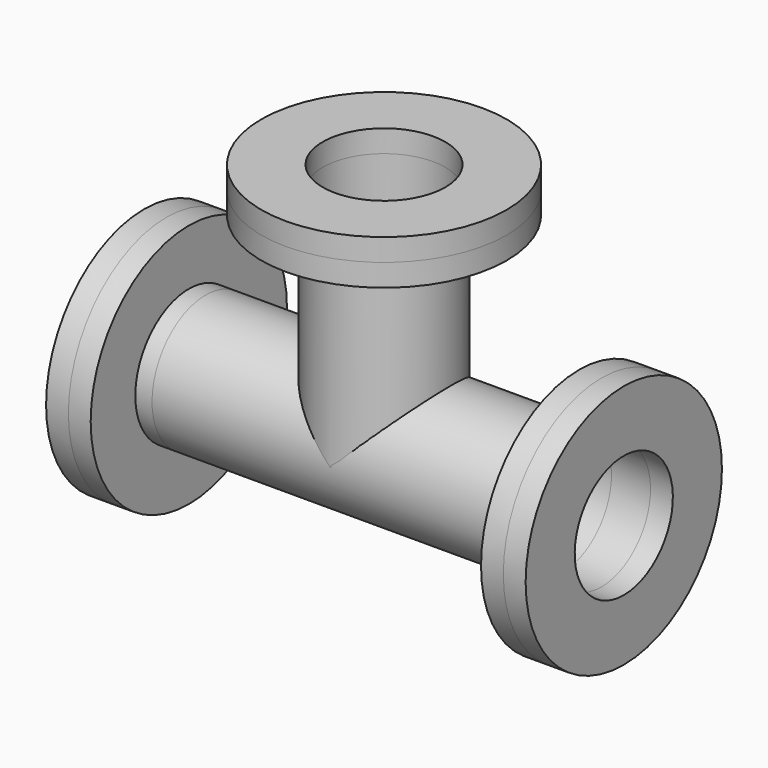
from build123d import *

# Parameters (mm, degrees)
F0_R      = 76.2
F0_R_2    = 69.85
F1_DEPTH  = 19.05
F2_R      = 139.7
F2_R_2    = 76.2
F2_R_3    = 69.85
F3_DEPTH  = 25.4
F9_ANGLE  = 90
F11_DEPTH = 406.4
F12_REACH = 558.4271469057
F13_DEPTH = 25.4
F14_DEPTH = 25.4
F15_DEPTH = 25.4


with BuildPart() as f1:
    # F0 (on Top) → F1 (new body)
    with BuildSketch(Plane.XY):
        Circle(F0_R)
        Circle(F0_R_2, mode=Mode.SUBTRACT)
    extrude(amount=F1_DEPTH)

    # F2 (on face) → F3 (join)
    with BuildSketch(Plane.XY.offset(19.05)):
        Circle(F2_R)
        Circle(F2_R_2, mode=Mode.SUBTRACT)
        Circle(F2_R_2)
        Circle(F2_R_3, mode=Mode.SUBTRACT)
    extrude(amount=F3_DEPTH)


with BuildPart() as f7_1:
    # F7: copy of F1
    add(f1.part.moved(Location((203.2, 0, -203.2))))


with BuildPart() as f7_1_1:
    # F9: moved
    add(f7_1.part.rotate(Axis((203.2, 122.1911609173, -203.2), (0, 1, 0)), F9_ANGLE))


with BuildPart() as f10_1:
    # F10: instance of F7_1
    add(f7_1_1.part.mirror(Plane.YZ))


with BuildPart() as f7_1_2:
    add(f7_1_1.part)

    # F11 (add, through all): a face of the model
    f11_faces = [f7_1_2.faces().sort_by_distance(p)[0] for p in [
        (203.2, 0, -129.1552614691),
    ]]

    add(f10_1.part)  # F11 merges F10_1
    extrude(f11_faces, amount=F11_DEPTH)


with BuildPart() as f1_1:
    add(f1.part)

    f12_end = f7_1_2.part.faces().sort_by_distance((0, 0, -127))[0]
    # F0 (on Top) → F12 (join, up to a face of F7_1 that its end follows)
    with BuildSketch(Plane.XY):
        Circle(F0_R)
        Circle(F0_R_2, mode=Mode.SUBTRACT)
    f12_long = extrude(amount=-F12_REACH, mode=Mode.PRIVATE)
    add(split(f12_long, bisect_by=f12_end, keep=Keep.ALL, mode=Mode.PRIVATE).solids().sort_by_distance((-74.0447385309, 0, 0))[0])


with BuildPart() as f13:
    # F13 (new): a face of the model
    f13_faces = [f1_1.part.faces().sort_by_distance(p)[0] for p in [
        (-135.7486873067, 0, 44.45),
    ]]
    extrude(f13_faces, amount=F13_DEPTH)


with BuildPart() as f14:
    # F14 (new): a face of the model
    f14_faces = [f7_1_2.part.faces().sort_by_distance(p)[0] for p in [
        (247.65, 0, -67.4513126933),
    ]]
    extrude(f14_faces, amount=F14_DEPTH)


with BuildPart() as f15:
    # F15 (new): a face of the model
    f15_faces = [f7_1_2.part.faces().sort_by_distance(p)[0] for p in [
        (-247.65, 0, -67.4513126933),
    ]]
    extrude(f15_faces, amount=F15_DEPTH)


solid = Compound([f7_1_2.part, f1_1.part, f13.part, f14.part, f15.part])
